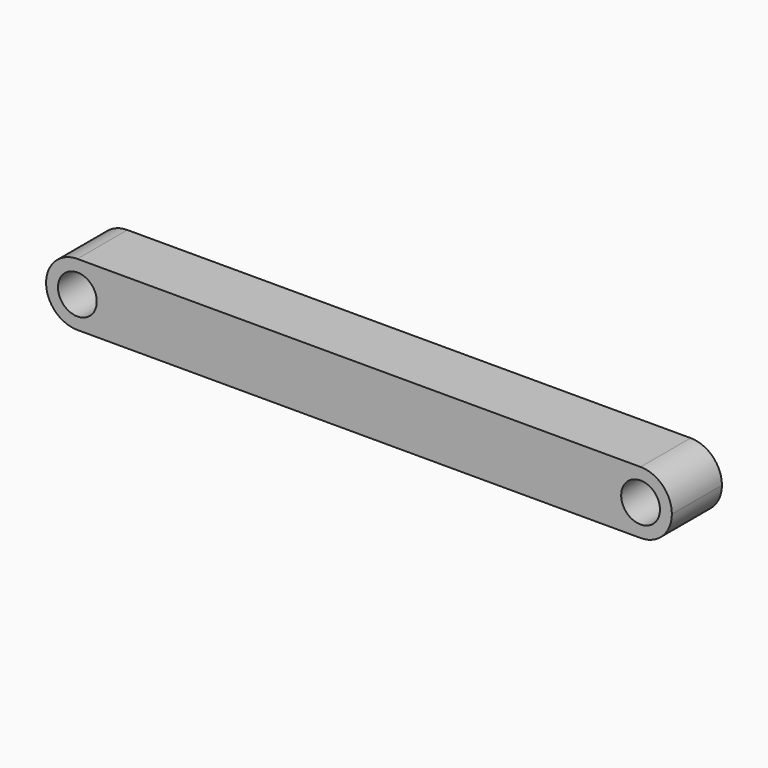
from build123d import *

# Parameters (mm, degrees)
F0_W     = 50
F0_H     = 5
F1_DEPTH = 2.5
F2_R     = 2.49999
F3_R     = 1.55
F4_DEPTH = 12.5


# Not quite as in the source:
# - a fillet or chamfer is up to 0.001 mm smaller than in the source, because OpenCascade refuses the exact size


with BuildPart() as f1:
    # F0 (on Front) → F1 (new body, symmetric)
    with BuildSketch(Plane.XZ):
        Rectangle(F0_W, F0_H)
    extrude(amount=F1_DEPTH, both=True)

    # F2 (radius 2.5 in the source; OpenCascade refuses exactly that, so slightly less here)
    f2_edges = [f1.edges().sort_by_distance(p)[0] for p in [
        (25, 0, 2.5),
        (25, 0, -2.5),
        (-25, 0, 2.5),
        (-25, 0, -2.5),
    ]]
    fillet(f2_edges, radius=F2_R)

    # F3 (on face) → F4 (cut, symmetric)
    with BuildSketch(Plane(origin=(0, 2.5, 0), x_dir=(-1, 0, 0), z_dir=(0, 1, 0))):
        with Locations((-22.5, 0)):
            Circle(F3_R)
        with Locations((22.5, 0)):
            Circle(F3_R)
    extrude(amount=F4_DEPTH, both=True, mode=Mode.SUBTRACT)


solid = f1.part
